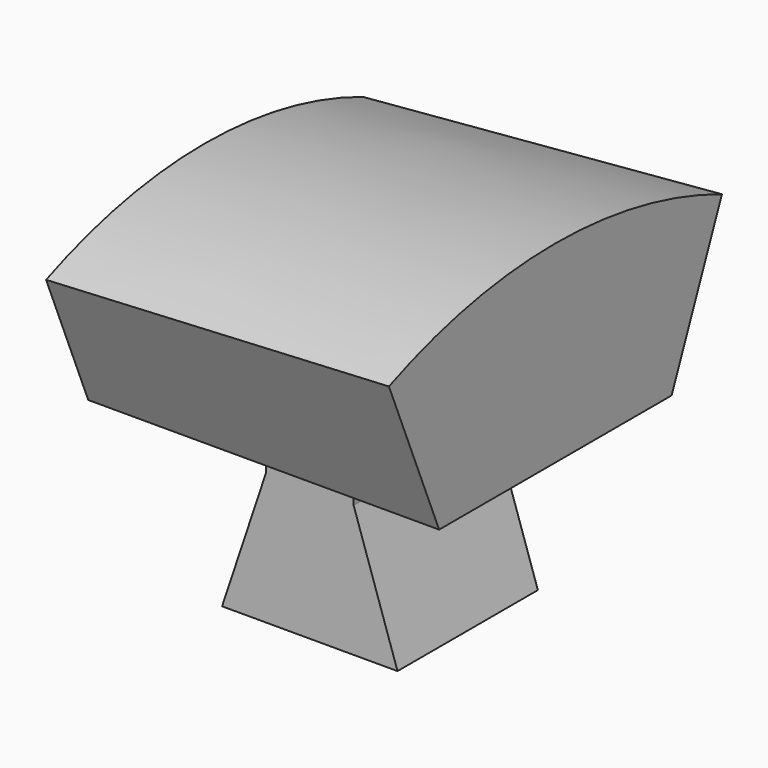
from build123d import *

# Parameters (mm, degrees)
F1_DEPTH      = 6.35
F2_ANGLE_BACK = 22.5
F2_ANGLE      = 45
F4_DEPTH      = 25.401
F5_DEPTH      = 2.54


with BuildPart() as f1:
    # F0 (on Front) → F1 (new body, symmetric)
    with BuildSketch(Plane.XZ):
        Polygon((-9.525, 22.1488), (-9.525, 25.4), (-15.875, 25.4), (-15.875, 22.1488), (-19.05, 12.6238), (-6.35, 12.6238), align=None)
    extrude(amount=F1_DEPTH, both=True)

    # F0 (on Front) → F2 (revolve)
    with BuildSketch(Plane.XZ, mode=Mode.PRIVATE) as f2_sk:
        Polygon((-9.525, 25.4), (0, 25.4), (0, 39.37), (-25.4, 37.465), (-25.4, 25.4), (-15.875, 25.4), align=None)
    revolve(f2_sk.sketch.rotate(Axis((-30.5623934027, 0, 0), (-1, 0, 0)), -F2_ANGLE_BACK), axis=Axis((-30.5623934027, 0, 0), (-1, 0, 0)), revolution_arc=F2_ANGLE)

    # F3 (on face) → F4 (cut, through all)
    with BuildSketch(Plane.YZ):
        with BuildLine():
            Line((11.3784447312, 25.4), (10.5210244843, 25.4))
            Line((10.5210244843, 25.4), (9.7201591821, 23.4665401258))
            ThreePointArc((9.7201591821, 23.4665401258), (4.9552941792, 24.9119461222), (0, 25.4))
            Line((0, 25.4), (0, 22.86))
            Line((0, 22.86), (11.3784447312, 22.86))
            Line((11.3784447312, 22.86), (11.3784447312, 25.4))
        make_face()
        with BuildLine():
            Line((9.7201591821, 23.4665401258), (10.5210244843, 25.4))
            Line((10.5210244843, 25.4), (0, 25.4))
            ThreePointArc((0, 25.4), (4.9552941792, 24.9119461222), (9.7201591821, 23.4665401258))
        make_face()
        with BuildLine():
            Line((0, 22.86), (0, 25.4))
            ThreePointArc((0, 25.4), (-4.9552941792, 24.9119461222), (-9.7201591821, 23.4665401258))
            Line((-9.7201591821, 23.4665401258), (-10.5210244843, 25.4))
            Line((-10.5210244843, 25.4), (-11.5035856143, 25.4))
            Line((-11.5035856143, 25.4), (-11.5035856143, 22.86))
            Line((-11.5035856143, 22.86), (0, 22.86))
        make_face()
        with BuildLine():
            ThreePointArc((-9.7201591821, 23.4665401258), (-4.9552941792, 24.9119461222), (0, 25.4))
            Line((0, 25.4), (-10.5210244843, 25.4))
            Line((-10.5210244843, 25.4), (-9.7201591821, 23.4665401258))
        make_face()
    extrude(amount=-F4_DEPTH, mode=Mode.SUBTRACT)

    # F5 (add, through all): a face of the model
    f5_faces = [f1.faces().sort_by_distance(p)[0] for p in [
        (-12.7, 0, 22.86),
    ]]
    extrude(f5_faces, amount=F5_DEPTH)


solid = f1.part
